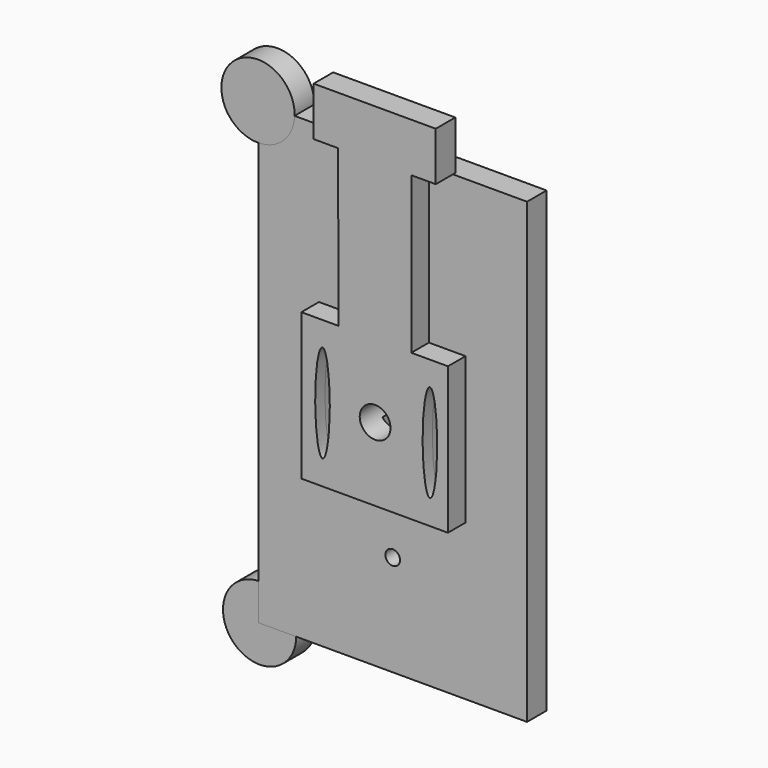
from build123d import *

# Parameters (mm, degrees)
F2_R     = 9.525
F3_DEPTH = 6.35
F0_W     = 69.85
F0_H     = 119.0625
F0_R     = 1.905
F0_W_2   = 6.35
F0_H_2   = 14.798598364
F0_R_2   = 1.8912469653
F1_R     = 9.525
F6_DEPTH = 3.175
F7_D     = 8.001


with BuildPart() as f3:
    # F2 (on Front) → F3 (new body)
    with BuildSketch(Plane.XZ):
        with Locations((-34.6031077206, -59.4968087971)):
            Circle(F2_R)
    extrude(amount=F3_DEPTH)


with BuildPart() as f3b:
    # F0 (on Front) → F3, piece 2 (new body)
    with BuildSketch(Plane.XZ):
        Rectangle(F0_W, F0_H)
        with Locations((0, -33.256188035)):
            Circle(F0_R, mode=Mode.SUBTRACT)
        Rectangle(F0_W_2, F0_H_2, mode=Mode.SUBTRACT)
        with Locations((0, 31.95521608)):
            Circle(F0_R_2, mode=Mode.SUBTRACT)
    extrude(amount=F3_DEPTH)

    # F5 (on face) → F6 (join, symmetric)
    with BuildSketch(Plane.XZ.offset(8.89)):
        Polygon((-15.9865934402, 59.6262310743), (-9.6336090937, 59.6260353923), (-9.5074940844, 18.9862310743), (-19.1689059138, 18.9862310743), (-19.1689059138, -19.1137689257), (18.9310940862, -19.1137689257), (18.9310940862, 18.9862310743), (9.4134065598, 18.9862310743), (9.4134065598, 59.6262310743), (15.7634065598, 59.6262310743), (15.7634065598, 72.3262310743), (-15.9865934402, 72.3262310743), align=None)
        with BuildLine():
            add(Edge.make_bspline(
                [(-13.6804133654, 12.7), (-16.9799701538, 12.7), (-15.3301917596, -6.35), (-13.6804133654, -25.4), (-12.0306349712, -6.35), (-10.3808565769, 12.7), (-13.6804133654, 12.7)],
                knots=[0, 0, 0, 2.0943951024, 2.0943951024, 4.1887902048, 4.1887902048, 6.2831853072, 6.2831853072, 6.2831853072], degree=2, weights=[1, 0.5, 1, 0.5, 1, 0.5, 1]))
        make_face(mode=Mode.SUBTRACT)
        with BuildLine():
            add(Edge.make_bspline(
                [(14.2465028912, 12.7), (10.9469461028, 12.7), (12.596724497, -6.35), (14.2465028912, -25.4), (15.8962812854, -6.35), (17.5460596796, 12.7), (14.2465028912, 12.7)],
                knots=[0, 0, 0, 2.0943951024, 2.0943951024, 4.1887902048, 4.1887902048, 6.2831853072, 6.2831853072, 6.2831853072], degree=2, weights=[1, 0.5, 1, 0.5, 1, 0.5, 1]))
        make_face(mode=Mode.SUBTRACT)
    extrude(amount=F6_DEPTH, both=True)

    # F7 (through all)
    with Locations(Plane(origin=(0, 0, 0), x_dir=(1, 0, 0), z_dir=(0, 1, 0))):
        with Locations((0, 0)):
            Hole(F7_D / 2)


with BuildPart() as f3c:
    # F1 (on Front) → F3, piece 3 (new body)
    with BuildSketch(Plane.XZ):
        with Locations((-35.0202806294, 59.8146952689)):
            Circle(F1_R)
    extrude(amount=F3_DEPTH)


solid = Compound([f3.part, f3b.part, f3c.part])
